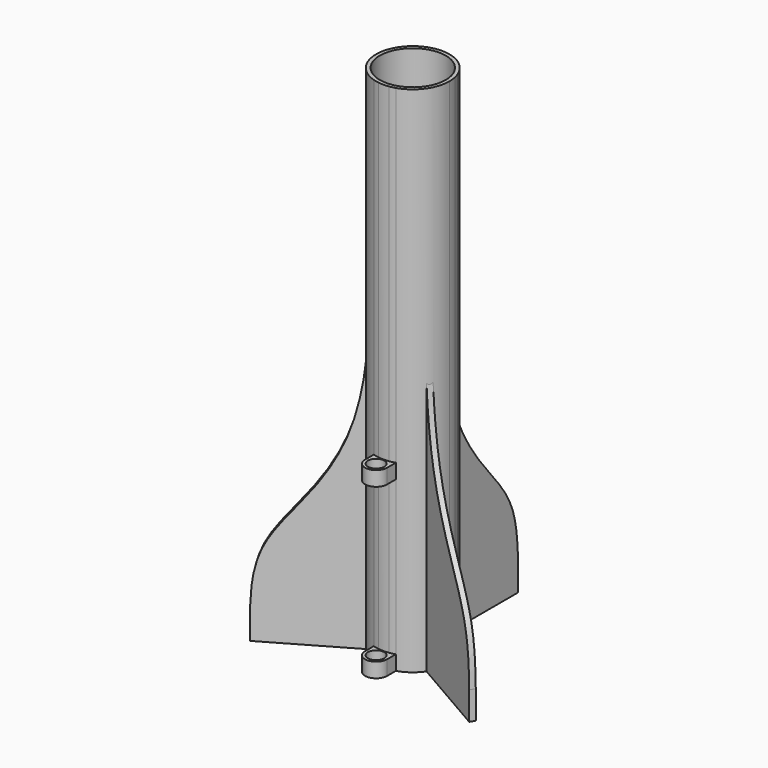
from build123d import *

# Parameters (mm, degrees)
F0_R      = 9
F1_DEPTH  = 140
F2_DEPTH  = 100
F4_DEPTH  = 10.751
F5_COUNT  = 3
F0_R_2    = 2.25
F6_DEPTH  = 4
F7_START  = 46
F7_DEPTH  = 4
F8_START  = 62
F0_R_3    = 7.5
F8_DEPTH  = 3
F10_DEPTH = 25


# Not quite as in the source:
# - a feature names something its author has since deleted; it is built from what else it names


with BuildPart() as f1:
    # F0 (on Top) → F1 (new body)
    with BuildSketch(Plane.XY):
        with BuildLine():
            ThreePointArc((-3, -9.5393920142), (-2.2464281062, -9.744411771), (-1.4791551643, -9.89))
            ThreePointArc((-1.4791551643, -9.89), (0, -10), (1.4791551643, -9.89))
            ThreePointArc((1.4791551643, -9.89), (2.2464281062, -9.744411771), (3, -9.5393920142))
            ThreePointArc((3, -9.5393920142), (8.0622577483, -5.9160797831), (10, 0))
            ThreePointArc((10, 0), (7.3314391493, 6.8007352544), (0.75, 9.9718353376))
            ThreePointArc((0.75, 9.9718353376), (0, 10), (-0.75, 9.9718353376))
            ThreePointArc((-0.75, 9.9718353376), (-9.9341644436, 1.1455901566), (-3, -9.5393920142))
        make_face()
        Circle(F0_R, mode=Mode.SUBTRACT)
    extrude(amount=F1_DEPTH)

    # F0 (on Top) → F2 (join)
    with BuildSketch(Plane.XY):
        with BuildLine():
            Line((-0.75, 34.9718353376), (-0.75, 9.9718353376))
            ThreePointArc((-0.75, 9.9718353376), (0, 10), (0.75, 9.9718353376))
            Line((0.75, 9.9718353376), (0.75, 34.9718353376))
            Line((0.75, 34.9718353376), (-0.75, 34.9718353376))
        make_face()
    extrude(amount=F2_DEPTH)

    # F3 (on face) → F4 (cut, through all)
    with BuildSketch(Plane.YZ.offset(0.75)):
        with BuildLine():
            Line((9.9718353376, 100), (9.9718353376, 75))
            Line((9.9718353376, 75), (9.9718353376, 69.1647440576))
            add(Edge.make_bspline(
                [(9.9718353376, 69.1647440576), (10.1832449594, 66.2204140215), (12.0836351221, 52.2918027042), (20.9708053433, 36.8272021249), (33.801245613, 23.6414831262), (34.7842815391, 13.599508776), (34.9718353376, 7.702038365)],
                knots=[0.0899218527, 0.0899218527, 0.0899218527, 0.0899218527, 0.2371904705, 0.3995520788, 0.5544857931, 0.7015059428, 0.7015059428, 0.7015059428, 0.7015059428], degree=3))
            Line((34.9718353376, 7.702038365), (34.9718353376, 100))
            Line((34.9718353376, 100), (9.9718353376, 100))
        make_face()
    extrude(amount=-F4_DEPTH, mode=Mode.SUBTRACT)


with BuildPart() as f5_1:
    # F5: instance of F1
    add(f1.part.rotate(Axis((0, 0, 0), (0, 0, 1)), 1 * 360 / F5_COUNT))


with BuildPart() as f5_2:
    # F5: instance of F1
    add(f1.part.rotate(Axis((0, 0, 0), (0, 0, 1)), 2 * 360 / F5_COUNT))


with BuildPart() as f1_1:
    add(f1.part)

    add(f5_1.part)  # F6 merges F5_1

    add(f5_2.part)  # F6 merges F5_2
    # F0 (on Top) → F6 (join)
    with BuildSketch(Plane.XY):
        with BuildLine():
            ThreePointArc((1.4791551643, -9.89), (0, -10), (-1.4791551643, -9.89))
            ThreePointArc((-1.4791551643, -9.89), (-2.592051841, -10.9896135416), (-3, -12.5))
            ThreePointArc((-3, -12.5), (0, -15.5), (3, -12.5))
            ThreePointArc((3, -12.5), (2.592051841, -10.9896135416), (1.4791551643, -9.89))
        make_face()
        with Locations((0, -12.5)):
            Circle(F0_R_2, mode=Mode.SUBTRACT)
        with BuildLine():
            ThreePointArc((-3, -12.5), (-2.592051841, -10.9896135416), (-1.4791551643, -9.89))
            ThreePointArc((-1.4791551643, -9.89), (-2.2464281062, -9.744411771), (-3, -9.5393920142))
            Line((-3, -9.5393920142), (-3, -12.5))
        make_face()
        with BuildLine():
            ThreePointArc((3, -9.5393920142), (2.2464281062, -9.744411771), (1.4791551643, -9.89))
            ThreePointArc((1.4791551643, -9.89), (2.592051841, -10.9896135416), (3, -12.5))
            Line((3, -12.5), (3, -9.5393920142))
        make_face()
    extrude(amount=F6_DEPTH)

    # F0 (on Top) → F7 (join)
    with BuildSketch(Plane.XY.offset(F7_START)):
        with BuildLine():
            ThreePointArc((1.4791551643, -9.89), (0, -10), (-1.4791551643, -9.89))
            ThreePointArc((-1.4791551643, -9.89), (-2.592051841, -10.9896135416), (-3, -12.5))
            ThreePointArc((-3, -12.5), (0, -15.5), (3, -12.5))
            ThreePointArc((3, -12.5), (2.592051841, -10.9896135416), (1.4791551643, -9.89))
        make_face()
        with Locations((0, -12.5)):
            Circle(F0_R_2, mode=Mode.SUBTRACT)
        with BuildLine():
            ThreePointArc((-3, -12.5), (-2.592051841, -10.9896135416), (-1.4791551643, -9.89))
            ThreePointArc((-1.4791551643, -9.89), (-2.2464281062, -9.744411771), (-3, -9.5393920142))
            Line((-3, -9.5393920142), (-3, -12.5))
        make_face()
        with BuildLine():
            ThreePointArc((3, -9.5393920142), (2.2464281062, -9.744411771), (1.4791551643, -9.89))
            ThreePointArc((1.4791551643, -9.89), (2.592051841, -10.9896135416), (3, -12.5))
            Line((3, -12.5), (3, -9.5393920142))
        make_face()
    extrude(amount=F7_DEPTH)

    # F0 (on Top) → F8 (join)
    with BuildSketch(Plane.XY.offset(F8_START)):
        Circle(F0_R)
        Circle(F0_R_3, mode=Mode.SUBTRACT)
    extrude(amount=F8_DEPTH)

    # F9 (on Front) → F10 (cut)
    with BuildSketch(Plane.XZ):
        with BuildLine():
            ThreePointArc((2.25, 115), (-1.5909902577, 116.5909902577), (0, 112.75))
            ThreePointArc((0, 112.75), (1.5909902577, 113.4090097423), (2.25, 115))
        make_face()
        with BuildLine():
            ThreePointArc((2.25, 103), (1.5909902577, 104.5909902577), (0, 105.25))
            ThreePointArc((0, 105.25), (-1.5909902577, 101.4090097423), (2.25, 103))
        make_face()
    extrude(amount=-F10_DEPTH, mode=Mode.SUBTRACT)


solid = f1_1.part
